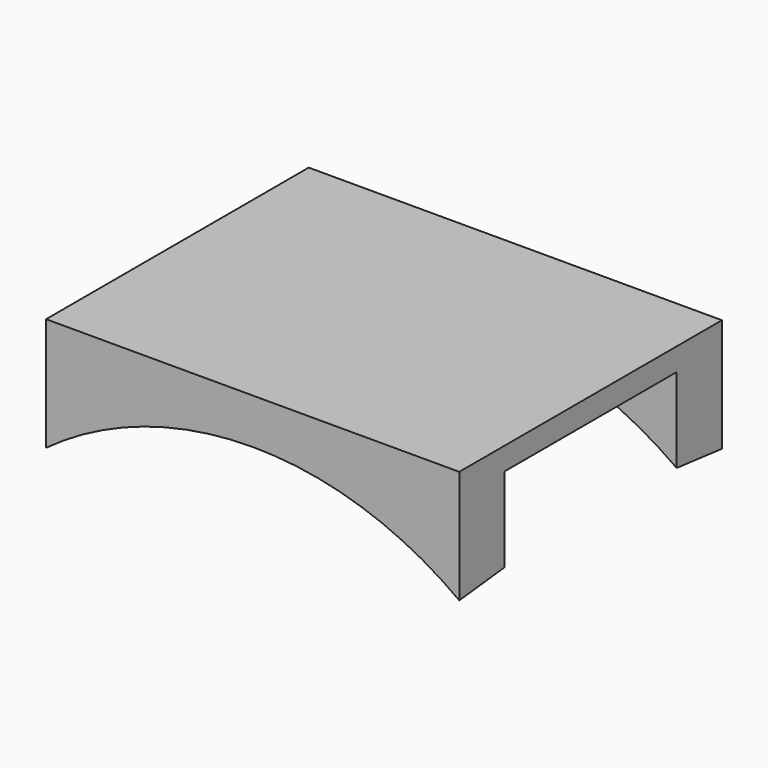
from build123d import *

# Parameters (mm, degrees)
F0_W       = 92.71
F0_H       = 73.66
F1_DEPTH   = 5.08
F2_W       = 92.71
F2_H       = 12.7
F3_DEPTH   = 20.32
F5_DEPTH   = 73.661
F6_SIZE2   = 1.111096
F6_SIZE    = 12.69999
F6_2_SIZE2 = 1.111096
F6_2_SIZE  = 12.69999


# Not quite as in the source:
# - a fillet or chamfer is up to 0.001 mm smaller than in the source, because OpenCascade refuses the exact size


with BuildPart() as f1:
    # F0 (on Top) → F1 (new body)
    with BuildSketch(Plane.XY):
        Rectangle(F0_W, F0_H)
    extrude(amount=F1_DEPTH)

    # F2 (on face) → F3 (join)
    with BuildSketch(Plane(origin=(0, 0, 0), x_dir=(1, 0, 0), z_dir=(0, 0, -1))):
        with Locations((0, 30.48)):
            Rectangle(F2_W, F2_H)
        with Locations((0, -30.48)):
            Rectangle(F2_W, F2_H)
    extrude(amount=F3_DEPTH)

    # F4 (on face) → F5 (cut, through all)
    with BuildSketch(Plane.XZ.offset(36.83)):
        with BuildLine():
            Line((-46.355, -20.32), (46.355, -20.32))
            ThreePointArc((46.355, -20.32), (0, -5.08), (-46.355, -20.32))
        make_face()
    extrude(amount=-F5_DEPTH, mode=Mode.SUBTRACT)

    # F6 (size 12.7 and 1.1111060268 in the source; OpenCascade refuses exactly that, so slightly less here)
    f6_edges = [f1.edges().sort_by_distance(p)[0] for p in [
        (0, 24.13, -5.08),
    ]]
    f6_side = f1.faces().sort_by_distance((0, 30.48, -5.08))[0]
    chamfer(f6_edges, length=F6_SIZE, length2=F6_SIZE2, reference=f6_side)

    # F6#2 (size 12.7 and 1.1111060268 in the source; OpenCascade refuses exactly that, so slightly less here)
    f6_2_edges = [f1.edges().sort_by_distance(p)[0] for p in [
        (0, -24.13, -5.08),
    ]]
    f6_2_side = f1.faces().sort_by_distance((0, -30.48, -5.08))[0]
    chamfer(f6_2_edges, length=F6_2_SIZE, length2=F6_2_SIZE2, reference=f6_2_side)


solid = f1.part
